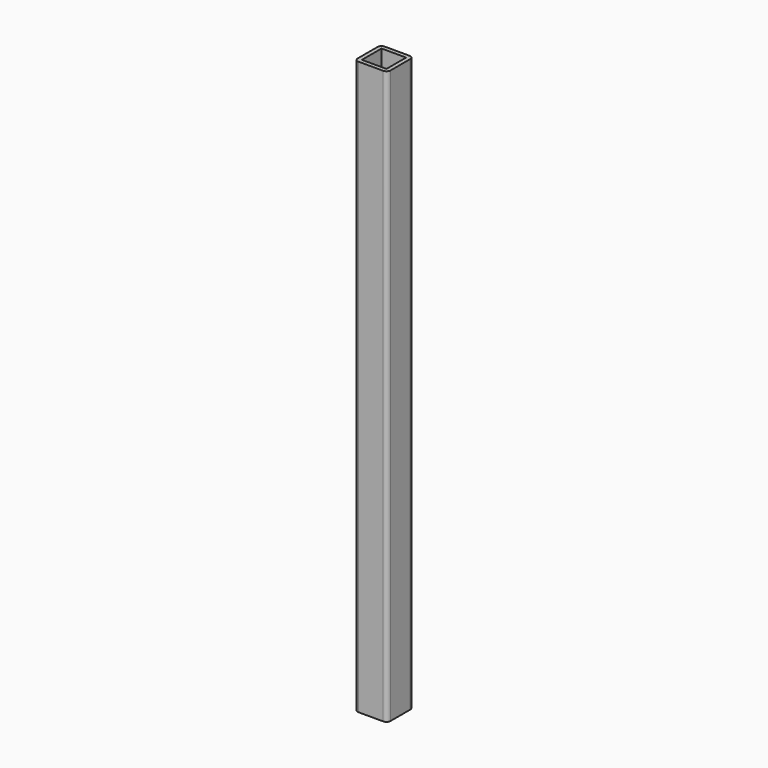
from build123d import *

# Parameters (mm, degrees)
F1_DEPTH = 889
F2_T     = 6.35


# Not quite as in the source:
# - a shell that OpenCascade refuses in one call is made with other operations: the cavity is built on its own and cut out


with BuildPart() as f1:
    # F0 (on Top) → F1 (new body)
    with BuildSketch(Plane.XY):
        with BuildLine():
            ThreePointArc((0, 6.35), (1.8598719395, 1.8598719395), (6.35, 0))
            Line((6.35, 0), (44.45, 0))
            ThreePointArc((44.45, 0), (48.9401280605, 1.8598719395), (50.8, 6.35))
            Line((50.8, 6.35), (50.8, 44.45))
            ThreePointArc((50.8, 44.45), (48.9401280605, 48.9401280605), (44.45, 50.8))
            Line((44.45, 50.8), (6.35, 50.8))
            ThreePointArc((6.35, 50.8), (1.8598719395, 48.9401280605), (0, 44.45))
            Line((0, 44.45), (0, 6.35))
        make_face()
    extrude(amount=F1_DEPTH)

    # F2: shell of thickness 6.35, made by hand


with BuildPart() as f2_core1:
    # F2_t2: copy of F1
    add(f1.part)

    # the walls: a layer under each face that stays
    f2_faces = [f2_core1.faces().sort_by_distance(p)[0] for p in [
        (0, 25.4, 444.5),
        (25.4, 0, 444.5),
        (50.8, 25.4, 444.5),
        (25.4, 50.8, 444.5),
    ]]
    thicken(f2_faces, amount=-F2_T, mode=Mode.SUBTRACT)


with BuildPart() as f1_1:
    add(f1.part)

    # what is left inside the walls is the cavity
    f2_cavity = [f2_core1.part.solids().sort_by_distance(p)[0] for p in [
        (6.4135, 25.4, 592.666667),
    ]]
    add(f2_cavity, mode=Mode.SUBTRACT)


solid = f1_1.part
